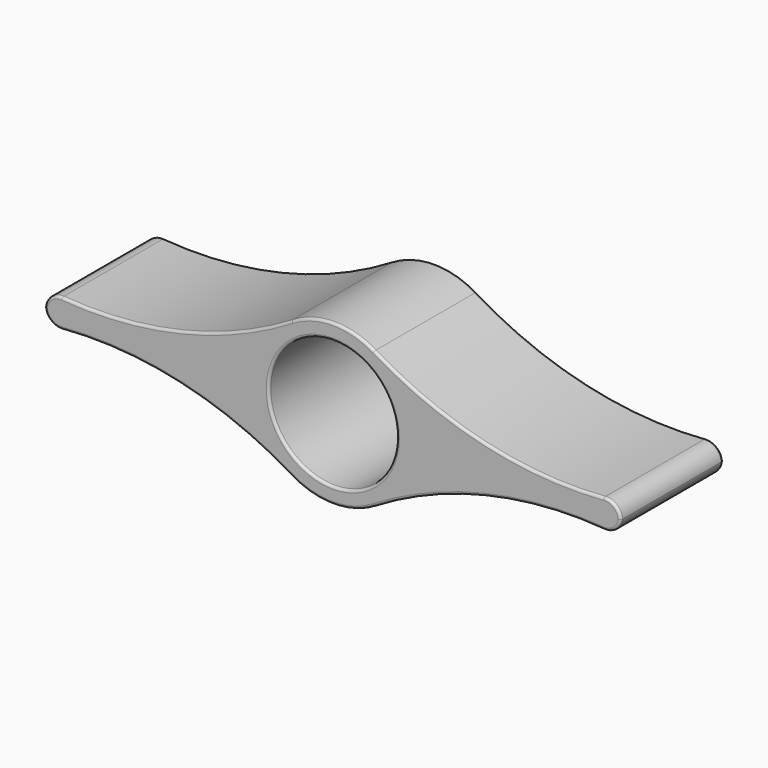
from build123d import *

# Parameters (mm, degrees)
F0_R        = 12.7
F1_DEPTH    = 25.4
F2_T1_DEPTH = 42.98370548
F3_R        = 0.508


# Not quite as in the source:
# - a fillet or chamfer that OpenCascade refuses, or shapes differently, is made with other operations: its cross-section is extruded or revolved along the edge and cut away or added


with BuildPart() as f1:
    # F0 (on Front) → F1 (new body)
    with BuildSketch(Plane.XZ):
        with BuildLine():
            ThreePointArc((-33.3693444663, 13.6158373531), (-27.7576647521, 19.4023003087), (-25.711236319, 27.1988529712))
            ThreePointArc((-25.711236319, 27.1988529712), (-27.7576647521, 34.9954056337), (-33.3693444663, 40.7818685893))
            ThreePointArc((-33.3693444663, 40.7818685893), (-41.586236319, 43.0738529712), (-49.8031281716, 40.7818685893))
            ThreePointArc((-49.8031281716, 40.7818685893), (-57.461236319, 27.1988529712), (-49.8031281716, 13.6158373531))
            ThreePointArc((-49.8031281716, 13.6158373531), (-41.586236319, 11.3238529712), (-33.3693444663, 13.6158373531))
        make_face()
        with Locations((-41.586236319, 27.1988529712)):
            Circle(F0_R, mode=Mode.SUBTRACT)
        with BuildLine():
            ThreePointArc((-33.3693444663, 40.7818685893), (-27.7576647521, 34.9954056337), (-25.711236319, 27.1988529712))
            ThreePointArc((-25.711236319, 27.1988529712), (-27.7576647521, 19.4023003087), (-33.3693444663, 13.6158373531))
            ThreePointArc((-33.3693444663, 13.6158373531), (-9.7812806597, 22.9500521891), (15.563763681, 24.0238529712))
            Line((15.563763681, 24.0238529712), (15.563763681, 27.1988529712))
            Line((15.563763681, 27.1988529712), (15.563763681, 30.3738529712))
            ThreePointArc((15.563763681, 30.3738529712), (-9.7812806597, 31.4476537533), (-33.3693444663, 40.7818685893))
        make_face()
        with BuildLine():
            ThreePointArc((-49.8031281716, 13.6158373531), (-57.461236319, 27.1988529712), (-49.8031281716, 40.7818685893))
            ThreePointArc((-49.8031281716, 40.7818685893), (-73.3911919783, 31.4476537533), (-98.736236319, 30.3738529712))
            Line((-98.736236319, 30.3738529712), (-98.736236319, 27.1988529712))
            Line((-98.736236319, 27.1988529712), (-98.736236319, 24.0238529712))
            ThreePointArc((-98.736236319, 24.0238529712), (-73.3911919783, 22.9500521891), (-49.8031281716, 13.6158373531))
        make_face()
    extrude(amount=F1_DEPTH)

    # F2: fillet of radius 3.175 on 4 edges, made by hand

    # F2_s2 → F2_t1 (cut)
    with BuildSketch(Plane.XZ.offset(-8.79185274)):
        with BuildLine():
            ThreePointArc((15.563763681, 26.8571118752), (14.5426395524, 29.1898021098), (12.1360825908, 30.0220411424))
            ThreePointArc((12.1360825908, 30.0220411424), (13.8519119629, 30.1785700373), (15.563763681, 30.3738529712))
            Line((15.563763681, 30.3738529712), (15.563763681, 26.8571118752))
        make_face()
        with BuildLine():
            ThreePointArc((12.1360825908, 24.3756648), (14.5426395524, 25.2079038326), (15.563763681, 27.5405940672))
            Line((15.563763681, 27.5405940672), (15.563763681, 24.0238529712))
            ThreePointArc((15.563763681, 24.0238529712), (13.8519119629, 24.219135905), (12.1360825908, 24.3756648))
        make_face()
        with BuildLine():
            ThreePointArc((-95.3085552288, 30.0220411424), (-97.7151121904, 29.1898021098), (-98.736236319, 26.8571118752))
            Line((-98.736236319, 26.8571118752), (-98.736236319, 30.3738529712))
            ThreePointArc((-98.736236319, 30.3738529712), (-97.0243846009, 30.1785700373), (-95.3085552288, 30.0220411424))
        make_face()
        with BuildLine():
            ThreePointArc((-98.736236319, 27.5405940672), (-97.7151121904, 25.2079038326), (-95.3085552288, 24.3756648))
            ThreePointArc((-95.3085552288, 24.3756648), (-97.0243846009, 24.219135905), (-98.736236319, 24.0238529712))
            Line((-98.736236319, 24.0238529712), (-98.736236319, 27.5405940672))
        make_face()
    extrude(amount=F2_T1_DEPTH, mode=Mode.SUBTRACT)

    # F3
    f3_edges = [f1.edges().sort_by_distance(p)[0] for p in [
        (-71.710097, -25.4, 31.825135),
        (-11.462375, 0, 31.825135),
        (-11.462375, -25.4, 22.572571),
        (-11.462375, 0, 22.572571),
        (-54.286236, -25.4, 27.198853),
        (-54.286236, 0, 27.198853),
    ]]
    fillet(f3_edges, radius=F3_R)


solid = f1.part
